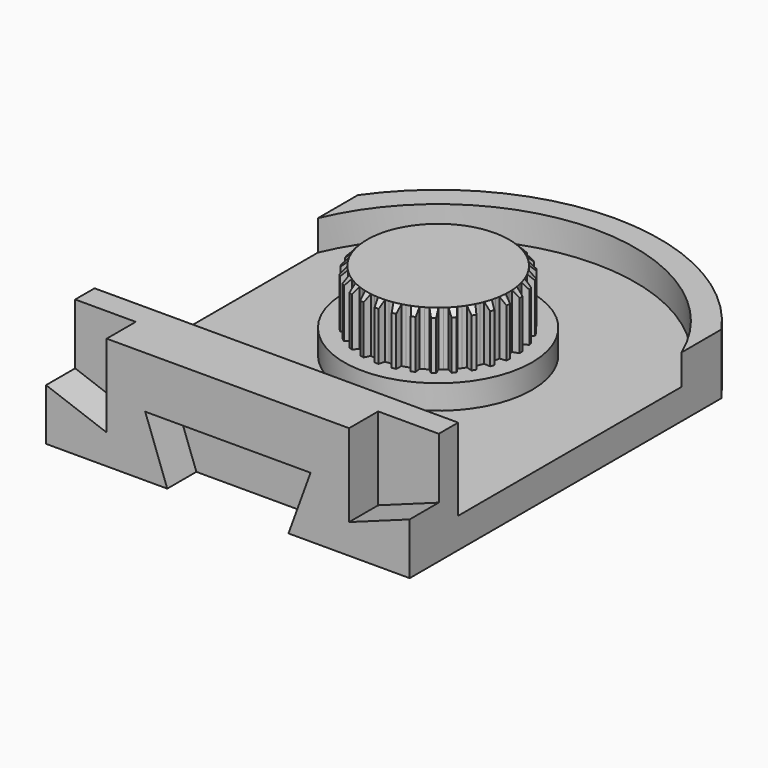
from build123d import *

# Parameters (mm, degrees)
F0_R            = 7.75
F1_DEPTH        = 2.5
F2_DEPTH        = 4.5
F3_DEPTH        = 9
F4_DEPTH        = 9.27
F5_SIZE         = 0.5
F6_START        = 4.5
F6_DEPTH        = 4.5
F6_COPIES_COUNT = 30
F8_W            = 10
F8_H            = 5
F8_W_2          = 5
F9_DEPTH        = 3
F10_DEPTH       = 5


# Not quite as in the source:
# - a feature of the source that left no trace in its solid (it failed there, or was rolled back) is left out
# - a pattern or mirror of a feature is missing from the dataset's text; its kind, count and spacing are read off the source's solid
# - a feature names something its author has since deleted; it is built from what else it names


with BuildPart() as f1:
    # F0 (on Top) → F1 (new body)
    with BuildSketch(Plane.XY):
        with BuildLine():
            ThreePointArc((15, 10.4610064645), (0, 18.2875), (-15, 10.4610064645))
            Line((-15, 10.4610064645), (-15, 6.3468619215))
            ThreePointArc((-15, 6.3468619215), (0, 16.2875), (15, 6.3468619215))
            Line((15, 6.3468619215), (15, 10.4610064645))
        make_face()
        with BuildLine():
            ThreePointArc((15, 6.3468619215), (0, 16.2875), (-15, 6.3468619215))
            Line((-15, 6.3468619215), (-15, -6.3468619215))
            ThreePointArc((-15, -6.3468619215), (0, -16.2875), (15, -6.3468619215))
            Line((15, -6.3468619215), (15, 6.3468619215))
        make_face()
        Circle(F0_R, mode=Mode.SUBTRACT)
        with BuildLine():
            ThreePointArc((-7.4806416837, -16.6875), (-11.663495105, -14.0852951047), (-15, -10.4610064645))
            Line((-15, -10.4610064645), (-15, -16.6875))
            Line((-15, -16.6875), (-7.4806416837, -16.6875))
        make_face()
        with BuildLine():
            Line((-15, -6.3468619215), (-15, -10.4610064645))
            ThreePointArc((-15, -10.4610064645), (-11.663495105, -14.0852951047), (-7.4806416837, -16.6875))
            Line((-7.4806416837, -16.6875), (7.4806416837, -16.6875))
            ThreePointArc((7.4806416837, -16.6875), (11.663495105, -14.0852951047), (15, -10.4610064645))
            Line((15, -10.4610064645), (15, -6.3468619215))
            ThreePointArc((15, -6.3468619215), (0, -16.2875), (-15, -6.3468619215))
        make_face()
        with BuildLine():
            Line((15, -16.6875), (15, -10.4610064645))
            ThreePointArc((15, -10.4610064645), (11.663495105, -14.0852951047), (7.4806416837, -16.6875))
            Line((7.4806416837, -16.6875), (15, -16.6875))
        make_face()
    extrude(amount=F1_DEPTH)

    # F0 (on Top) → F2 (join)
    with BuildSketch(Plane.XY):
        Circle(F0_R)
        with BuildLine():
            ThreePointArc((6.3302843538, 0.5), (6.345069174, 0.2501942779), (6.35, 0))
            ThreePointArc((6.35, 0), (6.345069174, -0.2501942779), (6.3302843538, -0.5))
            ThreePointArc((6.3302843538, -0.5), (-6.35, 0), (6.3302843538, 0.5))
        make_face(mode=Mode.SUBTRACT)
    extrude(amount=F2_DEPTH)

    # F0 (on Top) → F3 (join)
    with BuildSketch(Plane.XY):
        with BuildLine():
            Line((5.841133403, 0.3219636138), (6.3302843538, 0.5))
            ThreePointArc((6.3302843538, 0.5), (-6.35, 0), (6.3302843538, -0.5))
            Line((6.3302843538, -0.5), (5.841133403, -0.3219636138))
            ThreePointArc((5.841133403, -0.3219636138), (-5.85, 0), (5.841133403, 0.3219636138))
        make_face()
        with BuildLine():
            ThreePointArc((6.3302843538, -0.5), (6.345069174, -0.2501942779), (6.35, 0))
            ThreePointArc((6.35, 0), (6.345069174, 0.2501942779), (6.3302843538, 0.5))
            Line((6.3302843538, 0.5), (5.841133403, 0.3219636138))
            ThreePointArc((5.841133403, 0.3219636138), (5.8477829306, 0.1610428399), (5.85, 0))
            ThreePointArc((5.85, 0), (5.8477829306, -0.1610428399), (5.841133403, -0.3219636138))
            Line((5.841133403, -0.3219636138), (6.3302843538, -0.5))
        make_face()
        with BuildLine():
            ThreePointArc((5.85, 0), (5.8477829306, 0.1610428399), (5.841133403, 0.3219636138))
            ThreePointArc((5.841133403, 0.3219636138), (-5.85, 0), (5.841133403, -0.3219636138))
            ThreePointArc((5.841133403, -0.3219636138), (5.8477829306, -0.1610428399), (5.85, 0))
        make_face()
    extrude(amount=F3_DEPTH)

    # F0 (on Top) → F4 (join)
    with BuildSketch(Plane.XY):
        with BuildLine():
            Line((-7.4806416837, -16.6875), (-15, -16.6875))
            Line((-15, -16.6875), (-15, -21.6875008196))
            Line((-15, -21.6875008196), (15, -21.6875008196))
            Line((15, -21.6875008196), (15, -16.6875))
            Line((15, -16.6875), (7.4806416837, -16.6875))
            ThreePointArc((7.4806416837, -16.6875), (0, -18.2875), (-7.4806416837, -16.6875))
        make_face()
        with BuildLine():
            Line((7.4806416837, -16.6875), (-7.4806416837, -16.6875))
            ThreePointArc((-7.4806416837, -16.6875), (0, -18.2875), (7.4806416837, -16.6875))
        make_face()
    extrude(amount=F4_DEPTH)

    # F5
    f5_edges = [f1.edges().sort_by_distance(p)[0] for p in [
        (-6.330284, 0.5, 9),
    ]]
    chamfer(f5_edges, length=F5_SIZE)

    # F0 (on Top) → F6 (cut)
    with BuildSketch(Plane.XY.offset(F6_START)):
        with BuildLine():
            ThreePointArc((6.3302843538, -0.5), (6.345069174, -0.2501942779), (6.35, 0))
            ThreePointArc((6.35, 0), (6.345069174, 0.2501942779), (6.3302843538, 0.5))
            Line((6.3302843538, 0.5), (5.841133403, 0.3219636138))
            ThreePointArc((5.841133403, 0.3219636138), (5.8477829306, 0.1610428399), (5.85, 0))
            ThreePointArc((5.85, 0), (5.8477829306, -0.1610428399), (5.841133403, -0.3219636138))
            Line((5.841133403, -0.3219636138), (6.3302843538, -0.5))
        make_face()
    f6 = extrude(amount=F6_DEPTH, mode=Mode.SUBTRACT)

    # F6_copies: F6 ×30 about axis
    f6_copies_axis = Axis((0, 0, 0), (0, 0, 1))
    for i in range(1, F6_COPIES_COUNT):
        add(f6.rotate(f6_copies_axis, i * 360 / F6_COPIES_COUNT), mode=Mode.SUBTRACT)

    # F8 (on face) → F9 (cut)
    with BuildSketch(Plane.XZ.offset(21.6875008196)):
        Polygon((5, 5), (5, 0), (6.8198511713, 5), align=None)
        with Locations((0, 2.5)):
            Rectangle(F8_W, F8_H)
        Polygon((-6.8198511713, 5), (-5, 0), (-5, 5), align=None)
        with Locations((-12.5, 6.77)):
            Rectangle(F8_W_2, F8_H)
        Polygon((-10, 4.27), (-15, 4.27), (-10, 2.4501488287), align=None)
        Polygon((10, 2.4501488287), (15, 4.27), (15, 9.27), (10, 9.27), (10, 4.27), align=None)
    extrude(amount=-F9_DEPTH, mode=Mode.SUBTRACT)

    # F0 (on Top) → F10 (join)
    with BuildSketch(Plane.XY):
        with BuildLine():
            ThreePointArc((15, 10.4610064645), (0, 18.2875), (-15, 10.4610064645))
            Line((-15, 10.4610064645), (-15, 6.3468619215))
            ThreePointArc((-15, 6.3468619215), (0, 16.2875), (15, 6.3468619215))
            Line((15, 6.3468619215), (15, 10.4610064645))
        make_face()
    extrude(amount=F10_DEPTH)


solid = f1.part
